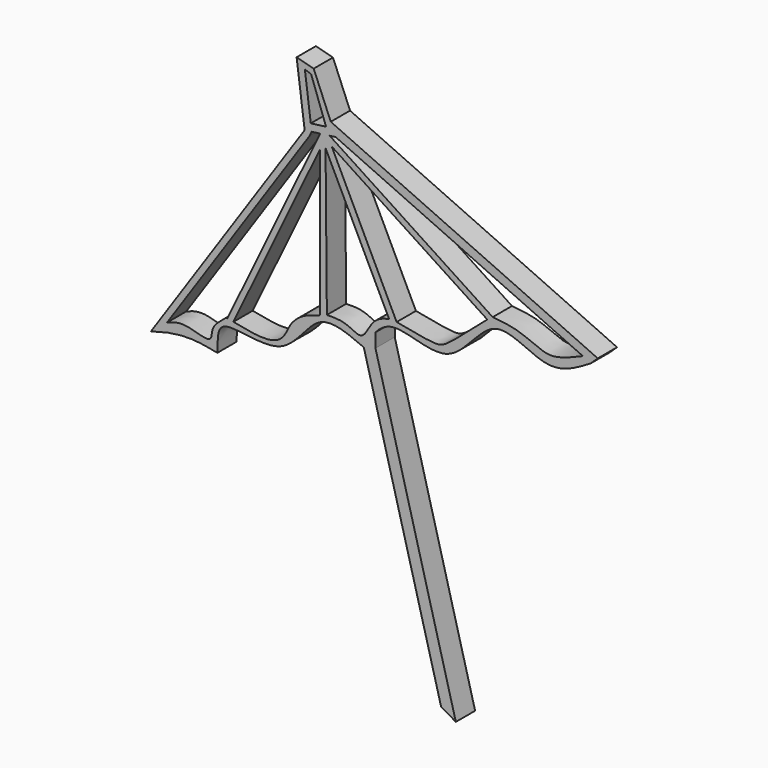
from build123d import *

# Parameters (mm, degrees)
F1_DEPTH    = 2
F2_T1_DEPTH = 27.7168298797


# Not quite as in the source:
# - a fillet or chamfer that OpenCascade refuses, or shapes differently, is made with other operations: its cross-section is extruded or revolved along the edge and cut away or added


with BuildPart() as f1:
    # F0 (on Front) → F1 (new body)
    with BuildSketch(Plane.XZ):
        with BuildLine():
            Line((38.9543399215, 33.578529954), (46.6473846136, 4.5816842054))
            Line((46.6473846136, 4.5816842054), (47.6139461386, 4.8381190285))
            Line((47.6139461386, 4.8381190285), (39.9209014464, 33.834964777))
            Line((39.9209014464, 33.834964777), (39.9209014464, 34.991762988))
            add(Edge.make_bspline(
                [(38.9543399215, 33.578529954), (39.261396009, 34.083414355), (39.5680450127, 34.5875702619), (39.9209014464, 34.991762988)],
                knots=[0, 0, 0, 0, 0.0840395323, 0.0840395323, 0.0840395323, 0.0840395323], degree=3))
        make_face()
        with BuildLine():
            add(Edge.make_bspline(
                [(38.9543399215, 33.578529954), (37.6640439923, 34.1443154), (34.8932435121, 35.3619439278), (32.5863528285, 29.9762581485), (26.5655761049, 32.3528079023), (26.8476535004, 30.0684064483), (26.7979316413, 29.2242113501)],
                knots=[0, 0, 0, 0, 0.2516937882, 0.52851586, 0.8089732942, 1, 1, 1, 1], degree=3))
            add(Edge.make_bspline(
                [(38.9543399215, 33.578529954), (39.261396009, 34.083414355), (39.5680450127, 34.5875702619), (39.9209014464, 34.991762988)],
                knots=[0, 0, 0, 0, 0.0840395323, 0.0840395323, 0.0840395323, 0.0840395323], degree=3))
            add(Edge.make_bspline(
                [(39.9209014464, 34.991762988), (40.305091024, 35.4318474469), (40.7440586925, 35.7534273237), (41.2979722023, 35.8284153044)],
                knots=[0.0840395323, 0.0840395323, 0.0840395323, 0.0840395323, 0.1755416542, 0.1755416542, 0.1755416542, 0.1755416542], degree=3))
            add(Edge.make_bspline(
                [(41.2979722023, 35.8284153044), (41.4906721415, 35.8545027334), (41.6972835341, 35.850746093), (41.914248864, 35.8273036468)],
                knots=[0.1755416542, 0.1755416542, 0.1755416542, 0.1755416542, 0.2073741569, 0.2073741569, 0.2073741569, 0.2073741569], degree=3))
            add(Edge.make_bspline(
                [(41.914248864, 35.8273036468), (43.1236682433, 35.696629549), (46.5485390265, 34.0361170247), (48.7293844979, 38.5978142218), (50.4905452243, 38.5674441057), (50.8079711977, 38.5090563461)],
                knots=[0.2073741569, 0.2073741569, 0.2073741569, 0.2073741569, 0.3848165425, 0.6042792737, 0.6509015915, 0.6509015915, 0.6509015915, 0.6509015915], degree=3))
            Line((50.8079711977, 38.5090563461), (49.6484453004, 39.2675593609))
            Line((49.6484453004, 39.2675593609), (36.1188769209, 48.1179165882))
            Line((36.1188769209, 48.1179165882), (36.6174241261, 48.182718962))
            Line((36.6174241261, 48.182718962), (57.1271326119, 38.8518427461))
            Line((57.1271326119, 38.8518427461), (57.7971301973, 38.5470278562))
            Line((57.7971301973, 38.5470278562), (58.3644174039, 39.0885546803))
            Line((58.3644174039, 39.0885546803), (36.2102526821, 49.1675750053))
            Line((36.2102526821, 49.1675750053), (34.7956053054, 52.5892884836))
            Line((34.7956053054, 52.5892884836), (33.3790388766, 52.9607144486))
            Line((33.3790388766, 52.9607144486), (34.0435805037, 47.848164531))
            Line((34.0435805037, 47.848164531), (21.2916761887, 29.0061510308))
            add(Edge.make_bspline(
                [(21.2916761887, 29.0061510308), (22.2377144422, 29.3003004789), (24.1919394004, 29.7248092747), (25.9431803037, 29.402753862), (26.7979316413, 29.2242113501)],
                knots=[0, 0, 0, 0, 0.5149489736, 1, 1, 1, 1], degree=3))
        make_face()
        with BuildLine():
            Line((35.3305023149, 48.0154417465), (27.6333307537, 32.0162793804))
            add(Edge.make_bspline(
                [(22.623414625, 30.0818228404), (23.0984624572, 30.271051787), (24.0718553407, 30.6285749561), (26.4700247065, 29.5668028622), (26.2229246754, 31.0093421737), (27.2691634193, 31.7917195395), (27.4724411863, 32.0150673015), (27.6333307537, 32.0162793804)],
                knots=[0, 0, 0, 0, 0.2344131875, 0.4959636953, 0.6719941358, 0.8783364267, 1, 1, 1, 1], degree=3))
            Line((22.623414625, 30.0818228404), (34.4592127341, 47.5702122015))
            Line((34.4592127341, 47.5702122015), (34.6295802641, 47.9243341999))
            Line((34.6295802641, 47.9243341999), (35.3305023149, 48.0154417465))
        make_face(mode=Mode.SUBTRACT)
        with BuildLine():
            add(Edge.make_bspline(
                [(28.1314488439, 31.9244866572), (28.7524146036, 31.8044131569), (30.0444740365, 31.5255182244), (31.7027687342, 31.5518548648), (32.4930864971, 32.4035579454), (32.8194445517, 33.3447504689), (33.7630925871, 34.2287315693), (34.7377791878, 34.5605212888), (35.1689763006, 34.6552392698), (35.3122933345, 34.7550361976)],
                knots=[0.0420238635, 0.0420238635, 0.0420238635, 0.0420238635, 0.1988600446, 0.3671317013, 0.4980303245, 0.6259677195, 0.7707900684, 0.901825209, 1, 1, 1, 1], degree=3))
            Line((28.1314488439, 31.9244866572), (35.3289500731, 46.8850458548))
            Line((35.3289500731, 46.8850458548), (35.3122933345, 34.7550361976))
        make_face(mode=Mode.SUBTRACT)
        with BuildLine():
            Line((35.7789325262, 47.0996380734), (41.0592946479, 36.3158529826))
            add(Edge.make_bspline(
                [(35.8884423072, 34.9503078622), (36.4754899607, 34.9773776718), (37.5532358859, 34.9460992821), (38.8819756802, 33.9391375769), (39.5472460755, 35.7321102048), (40.3992507331, 36.2208948371), (41.0592946479, 36.3158529826)],
                knots=[0, 0, 0, 0, 0.2672899311, 0.493356995, 0.7378410778, 1, 1, 1, 1], degree=3))
            Line((35.8884423072, 34.9503078622), (35.7789325262, 47.0996380734))
        make_face(mode=Mode.SUBTRACT)
        Polygon((35.8180012475, 48.678030682), (34.5529859469, 48.5136009278), (34.0623831223, 52.2879791273), (34.5787238251, 52.1228960279), align=None, mode=Mode.SUBTRACT)
        with BuildLine():
            add(Edge.make_bspline(
                [(41.6765891777, 36.3158529826), (42.8641978584, 36.0833171062), (44.6938094993, 35.7263694764), (45.6901446165, 35.8578817285), (47.6400405781, 37.6167605803), (48.6840130278, 38.4955786117), (49.1976533289, 38.9442550866)],
                knots=[0, 0, 0, 0, 0.305073377, 0.4728149529, 0.7460971216, 1, 1, 1, 1], degree=3))
            Line((41.6765891777, 36.3158529826), (36.2907871604, 47.3872721195))
            Line((36.2907871604, 47.3872721195), (49.1976533289, 38.9442550866))
        make_face(mode=Mode.SUBTRACT)
        with BuildLine():
            Line((49.6484453004, 39.2675593609), (50.8079711977, 38.5090563461))
            add(Edge.make_bspline(
                [(50.8079711977, 38.5090563461), (51.8830810784, 38.3112991915), (54.484160752, 36.5282918381), (56.6203789239, 37.8247061914), (57.7971301973, 38.5470278562)],
                knots=[0.6509015915, 0.6509015915, 0.6509015915, 0.6509015915, 0.8088096356, 1, 1, 1, 1], degree=3))
            Line((57.7971301973, 38.5470278562), (57.1271326119, 38.8518427461))
            add(Edge.make_bspline(
                [(49.6484453004, 39.2675593609), (50.3456305804, 39.2010948295), (51.7025455015, 39.0717365126), (53.4260999906, 38.2284905671), (54.784884825, 37.8599443173), (56.2669250792, 38.487560835), (57.1271326119, 38.8518427461)],
                knots=[0, 0, 0, 0, 0.2603727588, 0.5067572303, 0.7137114564, 1, 1, 1, 1], degree=3))
        make_face()
    extrude(amount=F1_DEPTH)

    # F2: chamfer of 5 on 1 edges, made by hand

    # F2_s2 → F2_t1 (cut)
    with BuildSketch(Plane.XZ.offset(-12.8584149398)):
        Polygon((45.3652104983, 9.4144918302), (51.4801922384, 5.8638583208), (46.6473846136, 4.5816842054), align=None)
    extrude(amount=F2_T1_DEPTH, mode=Mode.SUBTRACT)


solid = f1.part
